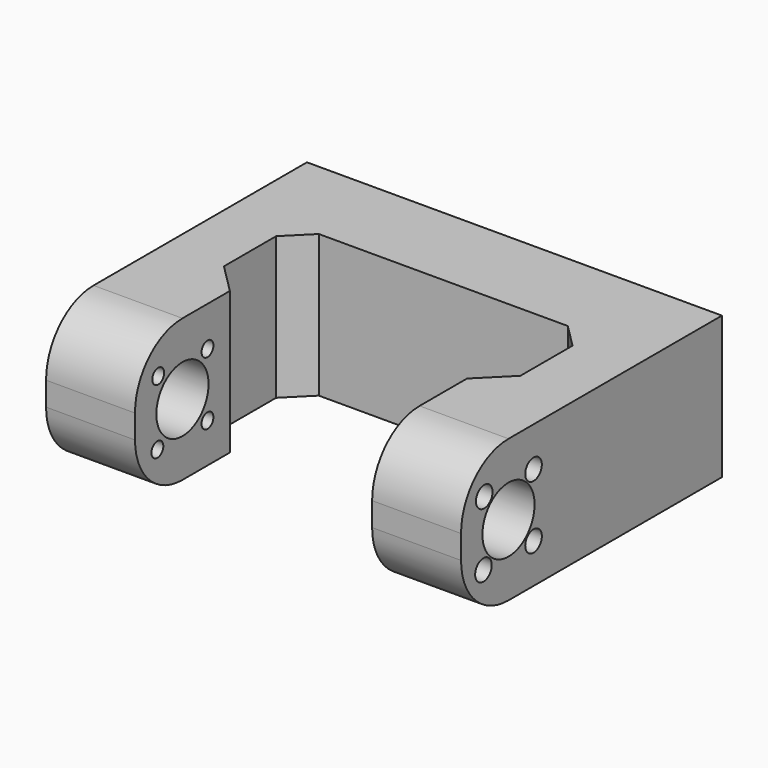
from build123d import *

# Parameters (mm, degrees)
F1_DEPTH       = 30.48
F4_D           = 13.97
F4_DEPTH       = 19.051
F4_ON_F2_D     = 13.97
F4_ON_F2_DEPTH = 19.051
F6_D           = 3.175
F8_SIZE        = 5.08
F9_SIZE        = 6.34999
F10_D          = 4.445
F10_DEPTH      = 12.7
F10_TIP        = 1.3354127258
F12_D          = 4.445
F12_DEPTH      = 12.7
F12_TIP        = 1.3354127258
F13_R          = 12.7


# Not quite as in the source:
# - a fillet or chamfer is up to 0.001 mm smaller than in the source, because OpenCascade refuses the exact size
# - a feature names something its author has since deleted; it is built from what else it names


with BuildPart() as f1:
    # F0 (on Top) → F1 (new body)
    with BuildSketch(Plane.XY):
        Polygon((38.1, 57.15), (-50.8, 57.15), (-50.8, -12.7), (-31.75, -12.7), (-31.75, 12.7), (-38.1, 12.7), (-38.1, 38.1), (25.4, 38.1), (25.4, 12.7), (19.05, 12.7), (19.05, -12.7), (38.1, -12.7), align=None)
    extrude(amount=F1_DEPTH)

    # F4 (through all, one way)
    with BuildSketch(Plane(origin=(19.05, 0, 0), x_dir=(0, -1, 0), z_dir=(-1, 0, 0))):
        with Locations((0, 15.24)):
            Circle(F4_D / 2)
    extrude(amount=-F4_DEPTH, mode=Mode.SUBTRACT)

    # F4 on F2 (through all, one way)
    with BuildSketch(Plane.YZ.offset(-31.75)):
        with Locations((0, 15.24)):
            Circle(F4_ON_F2_D / 2)
    extrude(amount=-F4_ON_F2_DEPTH, mode=Mode.SUBTRACT)

    # F6 (through all)
    with Locations(Plane(origin=(-50.8, 0, 0), x_dir=(0, -1, 0), z_dir=(-1, 0, 0))):
        with Locations((-6.706288951, 22.003272388), (6.4929844043, 22.2083615897), (6.706288951, 8.476727612), (-6.706288951, 8.476727612)):
            Hole(F6_D / 2)

    # F8
    f8_edges = [f1.edges().sort_by_distance(p)[0] for p in [
        (-38.1, 38.1, 15.24),
        (25.4, 38.1, 15.24),
    ]]
    chamfer(f8_edges, length=F8_SIZE)

    # F9 (size 6.35 in the source; OpenCascade refuses exactly that, so slightly less here)
    f9_edges = [f1.edges().sort_by_distance(p)[0] for p in [
        (25.4, 12.7, 15.24),
        (-38.1, 12.7, 15.24),
    ]]
    chamfer(f9_edges, length=F9_SIZE)

    # F10
    with Locations(Plane(origin=(-50.8, 0, 0), x_dir=(0, -1, 0), z_dir=(-1, 0, 0))):
        with Locations((6.4929844043, 22.2083615897), (6.706288951, 8.476727612), (-6.706288951, 8.476727612), (-6.706288951, 22.003272388)):
            Hole(F10_D / 2, depth=F10_DEPTH)
            with Locations((0, 0, -(F10_DEPTH + F10_TIP / 2))):  # 118° drill point
                Cone(0, F10_D / 2, F10_TIP, mode=Mode.SUBTRACT)

    # F12
    with Locations(Plane.YZ.offset(38.1)):
        with Locations((-6.706288951, 8.476727612), (-6.4929844043, 22.2083615897), (6.706288951, 22.003272388), (6.706288951, 8.476727612)):
            Hole(F12_D / 2, depth=F12_DEPTH)
            with Locations((0, 0, -(F12_DEPTH + F12_TIP / 2))):  # 118° drill point
                Cone(0, F12_D / 2, F12_TIP, mode=Mode.SUBTRACT)

    # F13
    f13_edges = [f1.edges().sort_by_distance(p)[0] for p in [
        (-41.275, -12.7, 30.48),
        (28.575, -12.7, 30.48),
        (28.575, -12.7, 0),
        (-41.275, -12.7, 0),
    ]]
    fillet(f13_edges, radius=F13_R)


solid = f1.part
